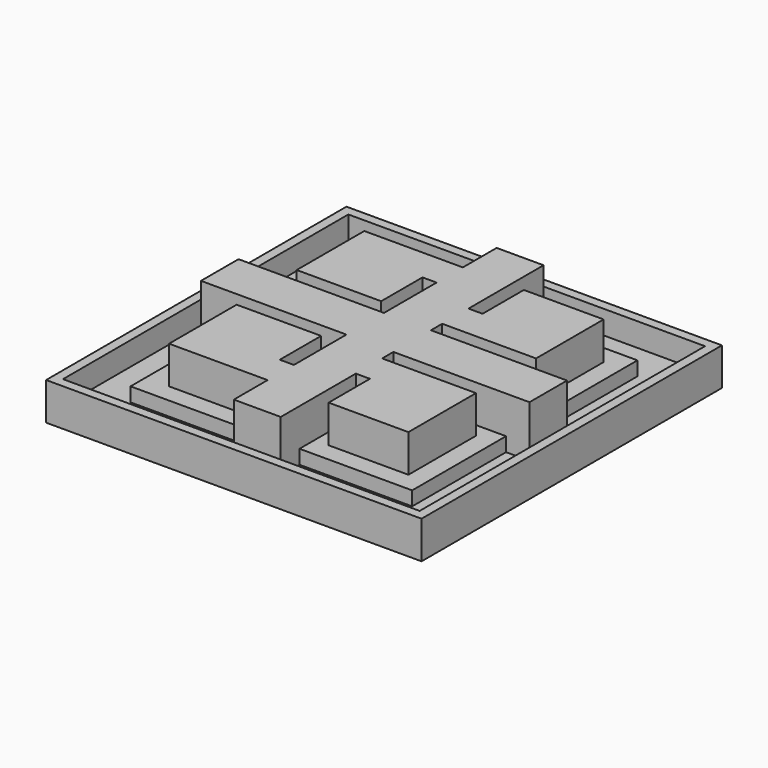
from build123d import *

# Parameters (mm, degrees)
F1_START = 3
F0_W     = 80
F0_H     = 80
F0_W_2   = 76
F0_H_2   = 76
F1_DEPTH = 51
F0_W_3   = 70
F0_H_3   = 70
F2_DEPTH = 3
F4_W     = 60
F4_H     = 60
F5_DEPTH = 3
F7_DEPTH = 5
F9_DEPTH = 11


# Not quite as in the source:
# - a pattern or mirror of a feature is missing from the dataset's text; its kind, count and spacing are read off the source's solid


with BuildPart() as f1:
    # F0 (on Top) → F1 (new body)
    with BuildSketch(Plane.XY.offset(F1_START)):
        Rectangle(F0_W, F0_H)
        Rectangle(F0_W_2, F0_H_2, mode=Mode.SUBTRACT)
    extrude(amount=F1_DEPTH)


with BuildPart() as f2:
    # F0 (on Top) → F2 (new body)
    with BuildSketch(Plane.XY):
        Rectangle(F0_W, F0_H)
        Rectangle(F0_W_2, F0_H_2, mode=Mode.SUBTRACT)
        Rectangle(F0_W_2, F0_H_2)
        Rectangle(F0_W_3, F0_H_3, mode=Mode.SUBTRACT)
        Rectangle(F0_W_3, F0_H_3)
    extrude(amount=-F2_DEPTH)

    # F4 (on Top) → F5 (join)
    with BuildSketch(Plane.XY):
        Rectangle(F4_W, F4_H)
    extrude(amount=F5_DEPTH)

    # F0 (on Top) → F7 (join)
    with BuildSketch(Plane.XY):
        Rectangle(F0_W, F0_H)
        Rectangle(F0_W_2, F0_H_2, mode=Mode.SUBTRACT)
    extrude(amount=F7_DEPTH)

    # F8 (on Top) → F9 (join)
    with BuildSketch(Plane.XY):
        Polygon((-35, 0), (35, 0), (35, 5), (6, 5), (6, 8), (26, 8), (26, 26), (9, 26), (9, 15), (6, 15), (6, 35), (-4, 35), (-4, 26), (-25, 26), (-25, 8), (-7, 8), (-7, 19), (-4, 19), (-4, 5), (-35, 5), align=None)
    f9 = extrude(amount=F9_DEPTH)

    # F9_copies: F9 across plane
    add(f9.mirror(Plane(origin=(0, 0, 0), x_dir=(0, 0, -1), z_dir=(0, -1, 0))))


solid = f2.part
